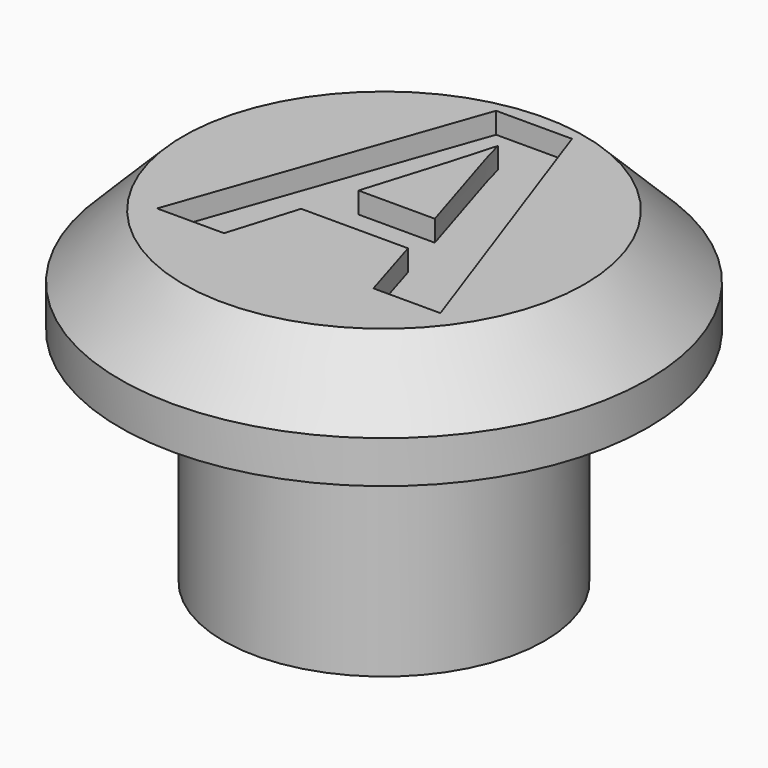
from build123d import *

# Parameters (mm, degrees)
F3_SIZE      = 3.81
F2_TEXT_SIZE = 24.6944444444
F5_DEPTH     = 1.27
F4_R         = 7.62
F6_DEPTH     = 12.7
F7_SIZE      = 1.27


# Not quite as in the source:
# - a feature names something its author has since deleted; it is built from what else it names
# - Text() gives the source's letters only with a copy of the font that has no kerning and outlines rounded to 1/6400 em; it was checked with that copy


with BuildPart() as f1:
    # F0 (on Front) → F1 (revolve)
    with BuildSketch(Plane.XZ):
        Polygon((0, 19.6714308113), (0, 0), (9.652, 0), (9.652, 13.3214308113), (15.875, 13.3214308113), (15.875, 19.6714308113), align=None)
    revolve(axis=Axis((0, 0, 7.2288028896), (0, 0, -1)))

    # F3
    f3_edges = [f1.edges().sort_by_distance(p)[0] for p in [
        (-15.875, 0, 19.671431),
    ]]
    chamfer(f3_edges, length=F3_SIZE)

    # F2 (on face) → F5 (cut)
    with BuildSketch(Plane.XY.offset(19.6714308113)):
        with Locations((-8.4299450266, -6.5224057184)):
            Text('A', F2_TEXT_SIZE, font='Open Sans', font_style=FontStyle.BOLD, text_align=(TextAlign.LEFT, TextAlign.BOTTOM))
    extrude(amount=-F5_DEPTH, mode=Mode.SUBTRACT)

    # F2 (on face) + F4 (on face) → F6 (cut)
    with BuildSketch(Plane.XY.offset(19.6714308113)):
        with Locations((-8.4299450266, -6.5224057184)):
            Text('A', F2_TEXT_SIZE, font='Open Sans', font_style=FontStyle.BOLD, text_align=(TextAlign.LEFT, TextAlign.BOTTOM))
    with BuildSketch(Plane(origin=(0, 0, 0), x_dir=(1, 0, 0), z_dir=(0, 0, -1))):
        Circle(F4_R)
    extrude(amount=F6_DEPTH, dir=(0, 0, 1), mode=Mode.SUBTRACT)

    # F7
    f7_edges = [f1.edges().sort_by_distance(p)[0] for p in [
        (-7.62, 0, 12.7),
    ]]
    chamfer(f7_edges, length=F7_SIZE)


solid = f1.part
